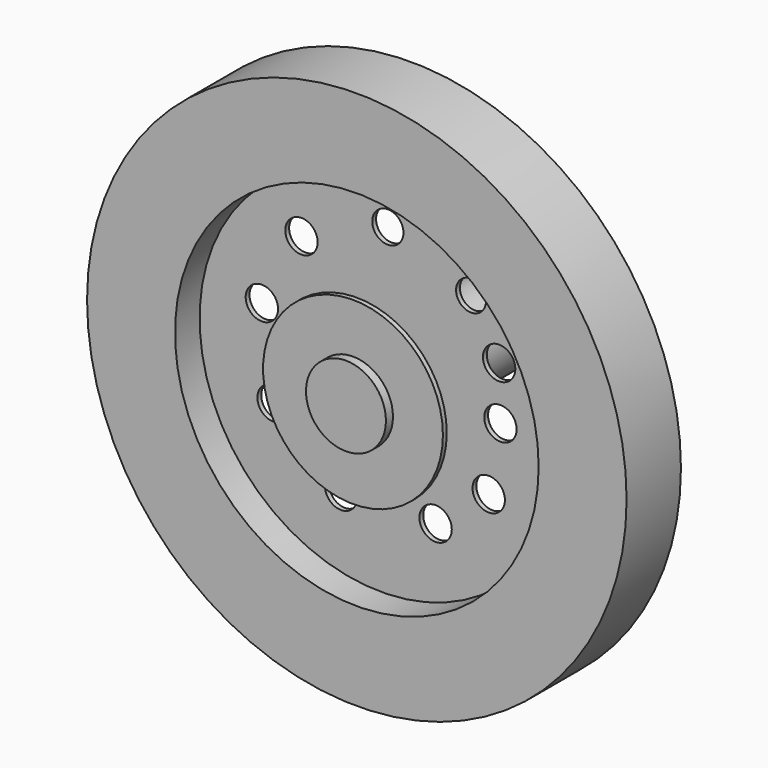
from build123d import *

# Parameters (mm, degrees)
F0_R      = 17.145
F1_DEPTH  = 4.318
F2_R      = 2.667
F3_DEPTH  = 9.7536
F4_R      = 2.54
F5_DEPTH  = 0.8636
F6_R      = 5.715
F7_DEPTH  = 0.3048
F8_R      = 11.557
F9_DEPTH  = 1.9558
F10_R     = 14.4638625387
F11_DEPTH = 0.508
F12_R     = 0.9919276493
F13_DEPTH = 35.4076
F14_R     = 11.557
F15_DEPTH = 1.5494
F18_R     = 0.9511664252
F19_DEPTH = 25.4
F20_R     = 1.0287
F21_DEPTH = 25.4
F22_R     = 1.0287
F23_DEPTH = 25.4


# Not quite as in the source:
# - the program builds the solid bodies; features that only make, move or delete a surface that nothing else refers to are left out


with BuildPart() as f1:
    # F0 (on Front) → F1 (new body)
    with BuildSketch(Plane.XZ):
        Circle(F0_R)
    extrude(amount=F1_DEPTH)

    # F2 (on Front) → F3 (join)
    with BuildSketch(Plane.XZ):
        Circle(F2_R)
    extrude(amount=-F3_DEPTH)

    # F4 (on face) → F5 (join)
    with BuildSketch(Plane.XZ.offset(4.318)):
        Circle(F4_R)
    extrude(amount=F5_DEPTH)

    # F6 (on face) → F7 (join)
    with BuildSketch(Plane.XZ.offset(4.318)):
        Circle(F6_R)
    extrude(amount=F7_DEPTH)

    # F8 (on face) → F9 (cut)
    with BuildSketch(Plane.XZ.offset(4.318)):
        Circle(F8_R)
    extrude(amount=-F9_DEPTH, mode=Mode.SUBTRACT)

    # F10 (on face) → F11 (cut)
    with BuildSketch(Plane.XZ.offset(2.3622)):
        Circle(F10_R)
    extrude(amount=-F11_DEPTH, mode=Mode.SUBTRACT)

    # F12 (on face) → F13 (cut)
    with BuildSketch(Plane.XZ.offset(4.318)):
        with Locations((0, 8.6582256481)):
            Circle(F12_R)
    extrude(amount=-F13_DEPTH, mode=Mode.SUBTRACT)

    # F14 (on face) → F15 (cut)
    with BuildSketch(Plane(origin=(0, 0, 0), x_dir=(-1, 0, 0), z_dir=(0, 1, 0))):
        Circle(F14_R)
    extrude(amount=-F15_DEPTH, mode=Mode.SUBTRACT)

    # F18 (on face) → F19 (cut)
    with BuildSketch(Plane.XZ.offset(4.318)):
        with Locations((5.286374595, 6.5436754376)):
            Circle(F18_R)
    extrude(amount=-F19_DEPTH, mode=Mode.SUBTRACT)

    # F20 (on face) → F21 (cut)
    with BuildSketch(Plane.XZ.offset(4.318)):
        with Locations((-8.0057960004, 1.8002251163)):
            Circle(F20_R)
        with Locations((-7.2620785795, -3.5718751606)):
            Circle(F20_R)
        with Locations((-2.9714044649, -7.1151754819)):
            Circle(F20_R)
        with Locations((3.035539994, -6.9437255152)):
            Circle(F20_R)
        with Locations((6.4108707011, -4.2005251162)):
            Circle(F20_R)
        with Locations((7.1545867249, 0)):
            Circle(F20_R)
        with Locations((7.0742800182, 3.3516884295)):
            Circle(F20_R)
    extrude(amount=-F21_DEPTH, mode=Mode.SUBTRACT)

    # F22 (on face) → F23 (cut)
    with BuildSketch(Plane.XZ.offset(4.318)):
        with Locations((-5.4886001162, 6.3565419987)):
            Circle(F22_R)
    extrude(amount=-F23_DEPTH, mode=Mode.SUBTRACT)


solid = f1.part
